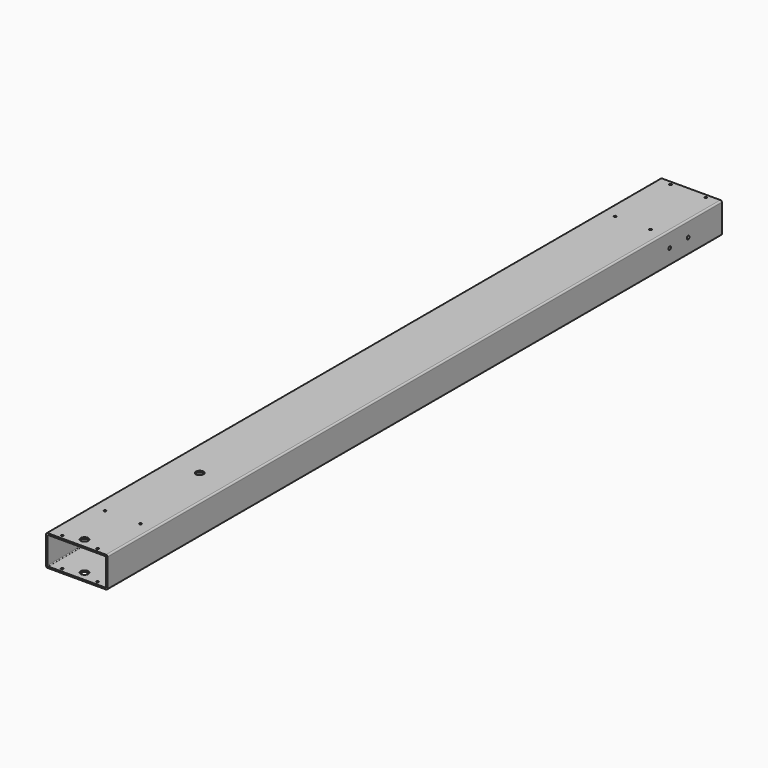
from build123d import *

# Parameters (mm, degrees)
F1_DEPTH  = 1000
F5_DEPTH  = 100
F7_DEPTH  = 100
F8_R      = 0.5
F8_2_R    = 0.5
F8_3_R    = 0.5
F8_4_R    = 0.5
F9_R      = 2.15
F10_DEPTH = 80.001
F11_R     = 1.5
F11_R_2   = 5
F12_DEPTH = 40.001


# Not quite as in the source:
# - a feature names something its author has since deleted; it is built from what else it names


with BuildPart() as f1:
    # F0 (on Front) → F1 (new body)
    with BuildSketch(Plane.XZ):
        with BuildLine():
            Line((38, 20), (-38, 20))
            ThreePointArc((-38, 20), (-39.4142135624, 19.4142135624), (-40, 18))
            Line((-40, 18), (-40, -18))
            ThreePointArc((-40, -18), (-39.4142135624, -19.4142135624), (-38, -20))
            Line((-38, -20), (38, -20))
            ThreePointArc((38, -20), (39.4142135624, -19.4142135624), (40, -18))
            Line((40, -18), (40, 18))
            ThreePointArc((40, 18), (39.4142135624, 19.4142135624), (38, 20))
        make_face()
        with BuildLine():
            ThreePointArc((-38, 17), (-37.7071067812, 17.7071067812), (-37, 18))
            Line((-37, 18), (37, 18))
            ThreePointArc((37, 18), (37.7071067812, 17.7071067812), (38, 17))
            Line((38, 17), (38, -17))
            ThreePointArc((38, -17), (37.7071067812, -17.7071067812), (37, -18))
            Line((37, -18), (-37, -18))
            ThreePointArc((-37, -18), (-37.7071067812, -17.7071067812), (-38, -17))
            Line((-38, -17), (-38, 17))
        make_face(mode=Mode.SUBTRACT)
    extrude(amount=F1_DEPTH)


with BuildPart() as f5:
    # F4 (on Front) → F5 (new body)
    with BuildSketch(Plane.XZ):
        with BuildLine():
            Line((36.5, 18), (-36.5, 18))
            ThreePointArc((-36.5, 18), (-37.5606601718, 17.5606601718), (-38, 16.5))
            ThreePointArc((-38, 16.5), (-37.5606601718, 15.4393398282), (-36.5, 15))
            Line((-36.5, 15), (36.5, 15))
            ThreePointArc((36.5, 15), (37.5606601718, 15.4393398282), (38, 16.5))
            ThreePointArc((38, 16.5), (37.5606601718, 17.5606601718), (36.5, 18))
        make_face()
    extrude(amount=F5_DEPTH)

    # F8
    f8_edges = [f5.edges().sort_by_distance(p)[0] for p in [
        (-23, -100, 15),
        (23, -100, 15),
        (0, -100, 18),
        (-38, -100, 16.5),
        (0, -100, 15),
        (38, -100, 16.5),
    ]]
    fillet(f8_edges, radius=F8_R)


with BuildPart() as f5b:
    # F4 (on Front) → F5, piece 2 (new body)
    with BuildSketch(Plane.XZ):
        with BuildLine():
            ThreePointArc((-38, -16.5), (-37.5606601718, -17.5606601718), (-36.5, -18))
            Line((-36.5, -18), (36.5, -18))
            ThreePointArc((36.5, -18), (37.5606601718, -17.5606601718), (38, -16.5))
            ThreePointArc((38, -16.5), (37.5606601718, -15.4393398282), (36.5, -15))
            Line((36.5, -15), (-36.5, -15))
            ThreePointArc((-36.5, -15), (-37.5606601718, -15.4393398282), (-38, -16.5))
        make_face()
    extrude(amount=F5_DEPTH)

    # F8#3
    f8_3_edges = [f5b.edges().sort_by_distance(p)[0] for p in [
        (-23, -100, -15),
        (23, -100, -15),
        (-38, -100, -16.5),
        (0, -100, -18),
        (38, -100, -16.5),
        (0, -100, -15),
    ]]
    fillet(f8_3_edges, radius=F8_3_R)


with BuildPart() as f7:
    # F6 (on Front) → F7 (new body)
    with BuildSketch(Plane.XZ):
        with BuildLine():
            Line((-10, 15), (-36, 15))
            ThreePointArc((-36, 15), (-37.4142135624, 14.4142135624), (-38, 13))
            Line((-38, 13), (-38, -13))
            ThreePointArc((-38, -13), (-37.4142135624, -14.4142135624), (-36, -15))
            Line((-36, -15), (-10, -15))
            ThreePointArc((-10, -15), (-8.5857864376, -14.4142135624), (-8, -13))
            Line((-8, -13), (-8, 13))
            ThreePointArc((-8, 13), (-8.5857864376, 14.4142135624), (-10, 15))
        make_face()
        with BuildLine():
            ThreePointArc((-36, 12), (-35.7071067812, 12.7071067812), (-35, 13))
            Line((-35, 13), (-11, 13))
            ThreePointArc((-11, 13), (-10.2928932188, 12.7071067812), (-10, 12))
            Line((-10, 12), (-10, -12))
            ThreePointArc((-10, -12), (-10.2928932188, -12.7071067812), (-11, -13))
            Line((-11, -13), (-35, -13))
            ThreePointArc((-35, -13), (-35.7071067812, -12.7071067812), (-36, -12))
            Line((-36, -12), (-36, 12))
        make_face(mode=Mode.SUBTRACT)
    extrude(amount=F7_DEPTH)

    # F8#2
    f8_2_edges = [f7.edges().sort_by_distance(p)[0] for p in [
        (-37.414214, -100, 14.414214),
        (-38, -100, 0),
        (-37.414214, -100, -14.414214),
        (-8.585786, -100, -14.414214),
        (-8, -100, 0),
        (-8.585786, -100, 14.414214),
        (-35.707107, -100, -12.707107),
        (-36, -100, 0),
        (-35.707107, -100, 12.707107),
        (-23, -100, 13),
        (-10.292893, -100, 12.707107),
        (-10, -100, 0),
        (-10.292893, -100, -12.707107),
        (-23, -100, -13),
    ]]
    fillet(f8_2_edges, radius=F8_2_R)


with BuildPart() as f7b:
    # F6 (on Front) → F7, piece 2 (new body)
    with BuildSketch(Plane.XZ):
        with BuildLine():
            ThreePointArc((10, 15), (8.5857864376, 14.4142135624), (8, 13))
            Line((8, 13), (8, -13))
            ThreePointArc((8, -13), (8.5857864376, -14.4142135624), (10, -15))
            Line((10, -15), (36, -15))
            ThreePointArc((36, -15), (37.4142135624, -14.4142135624), (38, -13))
            Line((38, -13), (38, 13))
            ThreePointArc((38, 13), (37.4142135624, 14.4142135624), (36, 15))
            Line((36, 15), (10, 15))
        make_face()
        with BuildLine():
            Line((35, -13), (11, -13))
            ThreePointArc((11, -13), (10.2928932188, -12.7071067812), (10, -12))
            Line((10, -12), (10, 12))
            ThreePointArc((10, 12), (10.2928932188, 12.7071067812), (11, 13))
            Line((11, 13), (35, 13))
            ThreePointArc((35, 13), (35.7071067812, 12.7071067812), (36, 12))
            Line((36, 12), (36, -12))
            ThreePointArc((36, -12), (35.7071067812, -12.7071067812), (35, -13))
        make_face(mode=Mode.SUBTRACT)
    extrude(amount=F7_DEPTH)

    # F8#4
    f8_4_edges = [f7b.edges().sort_by_distance(p)[0] for p in [
        (8.585786, -100, 14.414214),
        (8, -100, 0),
        (8.585786, -100, -14.414214),
        (37.414214, -100, -14.414214),
        (38, -100, 0),
        (37.414214, -100, 14.414214),
        (23, -100, -13),
        (10.292893, -100, -12.707107),
        (10, -100, 0),
        (10.292893, -100, 12.707107),
        (23, -100, 13),
        (35.707107, -100, 12.707107),
        (36, -100, 0),
        (35.707107, -100, -12.707107),
    ]]
    fillet(f8_4_edges, radius=F8_4_R)


with BuildPart() as f10_tool:
    # F9 (on face) → F10 (new body, through all)
    with BuildSketch(Plane.YZ.offset(40)):
        with Locations((-85, 0)):
            Circle(F9_R)
        with Locations((-55, 0)):
            Circle(F9_R)
    extrude(amount=-F10_DEPTH)


with BuildPart() as f1_1:
    add(f1.part)

    # F10: cut by f10_tool
    add(f10_tool.part, mode=Mode.SUBTRACT)


with BuildPart() as f7_1:
    add(f7.part)

    # F10: cut by f10_tool
    add(f10_tool.part, mode=Mode.SUBTRACT)


with BuildPart() as f7b_1:
    add(f7b.part)

    # F10: cut by f10_tool
    add(f10_tool.part, mode=Mode.SUBTRACT)


with BuildPart() as f12_tool:
    # F11 (on face) → F12 (new body, through all)
    with BuildSketch(Plane.XY.offset(20)):
        with Locations((-23, -5)):
            Circle(F11_R)
        with Locations((23, -5)):
            Circle(F11_R)
        with Locations((23, -95)):
            Circle(F11_R)
        with Locations((-23, -95)):
            Circle(F11_R)
        with Locations((-23, -925)):
            Circle(F11_R)
        with Locations((23, -925)):
            Circle(F11_R)
        with Locations((-23, -995)):
            Circle(F11_R)
        with Locations((23, -995)):
            Circle(F11_R)
        with Locations((0, -800)):
            Circle(F11_R_2)
        with Locations((0, -987.5)):
            Circle(F11_R_2)
    extrude(amount=-F12_DEPTH)


with BuildPart() as f1_2:
    add(f1_1.part)

    # F12: cut by f12_tool
    add(f12_tool.part, mode=Mode.SUBTRACT)


with BuildPart() as f5_1:
    add(f5.part)

    # F12: cut by f12_tool
    add(f12_tool.part, mode=Mode.SUBTRACT)


with BuildPart() as f5b_1:
    add(f5b.part)

    # F12: cut by f12_tool
    add(f12_tool.part, mode=Mode.SUBTRACT)


with BuildPart() as f7_2:
    add(f7_1.part)

    # F12: cut by f12_tool
    add(f12_tool.part, mode=Mode.SUBTRACT)


with BuildPart() as f7b_2:
    add(f7b_1.part)

    # F12: cut by f12_tool
    add(f12_tool.part, mode=Mode.SUBTRACT)


solid = Compound([f1_2.part, f5_1.part, f5b_1.part, f7_2.part, f7b_2.part])
